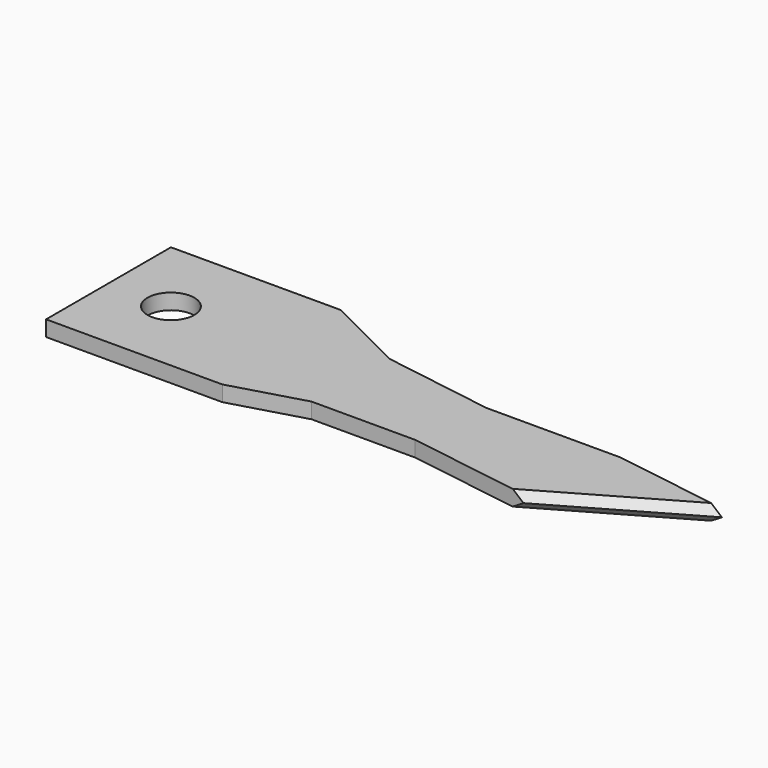
from build123d import *

# Parameters (mm, degrees)
F0_W        = 50.8
F0_H        = 12.7
F1_DEPTH    = 1.27
F2_R        = 1.905
F3_DEPTH    = 25.4
F5_DEPTH    = 25.4
F6_T1_DEPTH = 19.2858275148


# Not quite as in the source:
# - a fillet or chamfer that OpenCascade refuses, or shapes differently, is made with other operations: its cross-section is extruded or revolved along the edge and cut away or added


with BuildPart() as f1:
    # F0 (on Top) → F1 (new body)
    with BuildSketch(Plane.XY):
        with Locations((43.457204476, -21.0564464647)):
            Rectangle(F0_W, F0_H)
    extrude(amount=F1_DEPTH)

    # F2 (on face) → F3 (cut)
    with BuildSketch(Plane.XY.offset(1.27)):
        with Locations((23.137204476, -21.0564464647)):
            Circle(F2_R)
    extrude(amount=-F3_DEPTH, mode=Mode.SUBTRACT)

    # F4 (on face) → F5 (cut)
    with BuildSketch(Plane.XY.offset(1.27)):
        Polygon((58.4226325154, -19.4466076791), (68.857204476, -21.0564464647), (68.857204476, -14.7064464647), (31.86333552, -14.7064464647), (38.4808033705, -18.0158037692), (47.5127547979, -19.4466076791), align=None)
        Polygon((68.857204476, -27.4064464647), (68.857204476, -21.0564464647), (57.7966570854, -27.4064464647), align=None)
        Polygon((32.3998853564, -27.4064464647), (57.7966570854, -27.4064464647), (46.7079244554, -25.7063750178), (38.3019521832, -25.7063750178), align=None)
    extrude(amount=-F5_DEPTH, mode=Mode.SUBTRACT)

    # F6: chamfer of 1.27 on 2 edges, made by hand

    # F6_s2 → F6_t1 (cut)
    with BuildSketch(Plane(origin=(45.5281359874, 26.1382780897, 0), x_dir=(0, 0, 1), z_dir=(-0.8672386574, -0.4978926702, 0))):
        Polygon((1.27, -51.2744617638), (0, -52.5444617638), (1.27, -52.5444617638), align=None)
        Polygon((0, -51.2744617638), (1.27, -52.5444617638), (0, -52.5444617638), align=None)
    extrude(amount=F6_T1_DEPTH, mode=Mode.SUBTRACT)


solid = f1.part
